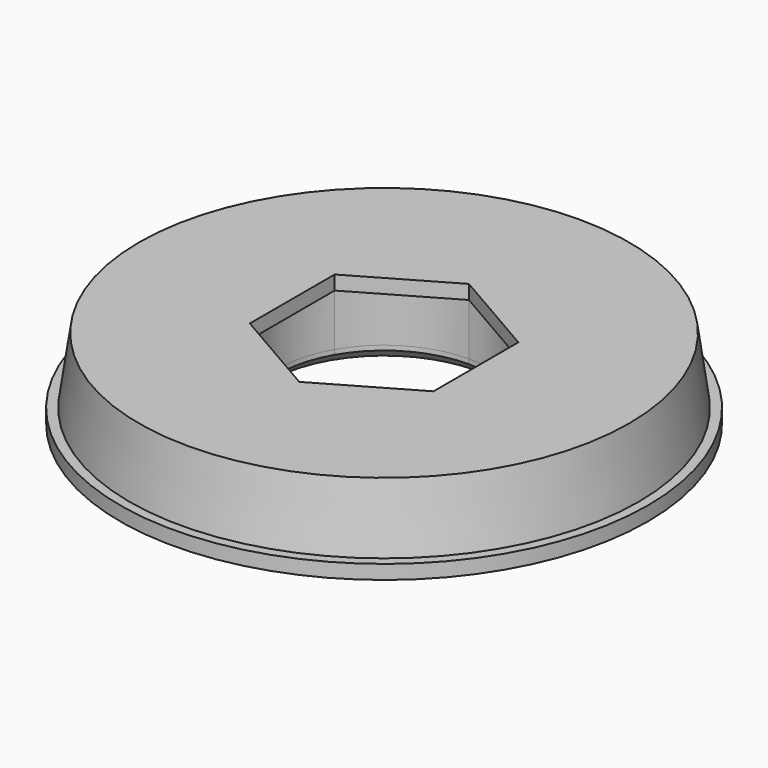
from build123d import *

# Parameters (mm, degrees)
F5_R          = 27
F6_DEPTH      = 7
F5_R_2        = 28
F7_DEPTH      = 1.5
F8_DEPTH      = 7.001
F8_DEPTH_BACK = 1.501
F9_DEPTH      = 5.5
F9_DEPTH_BACK = 1.501
F10_SIZE2     = 0.99999
F10_SIZE      = 6.99999
F11_SIZE      = 1


# Not quite as in the source:
# - a fillet or chamfer is up to 0.001 mm smaller than in the source, because OpenCascade refuses the exact size


with BuildPart() as f6:
    # F5 (on Top) → F6 (new body)
    with BuildSketch(Plane.XY):
        Circle(F5_R)
        with BuildLine():
            ThreePointArc((9.7427857926, 5.625), (10.8666655458, 2.9117142574), (11.25, 0))
            ThreePointArc((11.25, 0), (10.8666655458, -2.9117142574), (9.7427857926, -5.625))
            ThreePointArc((9.7427857926, -5.625), (5.625, -9.7427857926), (0, -11.25))
            ThreePointArc((0, -11.25), (-5.625, -9.7427857926), (-9.7427857926, -5.625))
            ThreePointArc((-9.7427857926, -5.625), (-11.25, 0), (-9.7427857926, 5.625))
            ThreePointArc((-9.7427857926, 5.625), (-5.625, 9.7427857926), (0, 11.25))
            ThreePointArc((0, 11.25), (5.625, 9.7427857926), (9.7427857926, 5.625))
        make_face(mode=Mode.SUBTRACT)
        with BuildLine():
            Line((-9.7427857926, -5.625), (-9.7427857926, 5.625))
            ThreePointArc((-9.7427857926, 5.625), (-11.25, 0), (-9.7427857926, -5.625))
        make_face()
        with BuildLine():
            Line((0, 11.25), (9.7427857926, 5.625))
            ThreePointArc((9.7427857926, 5.625), (5.625, 9.7427857926), (0, 11.25))
        make_face()
        with BuildLine():
            ThreePointArc((9.7427857926, -5.625), (10.8666655458, -2.9117142574), (11.25, 0))
            ThreePointArc((11.25, 0), (10.8666655458, 2.9117142574), (9.7427857926, 5.625))
            Line((9.7427857926, 5.625), (9.7427857926, -5.625))
        make_face()
        with BuildLine():
            ThreePointArc((0, -11.25), (5.625, -9.7427857926), (9.7427857926, -5.625))
            Line((9.7427857926, -5.625), (0, -11.25))
        make_face()
        with BuildLine():
            ThreePointArc((-9.7427857926, -5.625), (-5.625, -9.7427857926), (0, -11.25))
            Line((0, -11.25), (-9.7427857926, -5.625))
        make_face()
        with BuildLine():
            Line((-9.7427857926, 5.625), (0, 11.25))
            ThreePointArc((0, 11.25), (-5.625, 9.7427857926), (-9.7427857926, 5.625))
        make_face()
        Polygon((9.7427857926, -5.625), (9.7427857926, 5.625), (0, 11.25), (-9.7427857926, 5.625), (-9.7427857926, -5.625), (0, -11.25), align=None)
    extrude(amount=F6_DEPTH)

    # F5 (on Top) → F7 (join)
    with BuildSketch(Plane.XY):
        Circle(F5_R_2)
        Circle(F5_R, mode=Mode.SUBTRACT)
        Circle(F5_R)
        with BuildLine():
            ThreePointArc((9.7427857926, 5.625), (10.8666655458, 2.9117142574), (11.25, 0))
            ThreePointArc((11.25, 0), (10.8666655458, -2.9117142574), (9.7427857926, -5.625))
            ThreePointArc((9.7427857926, -5.625), (5.625, -9.7427857926), (0, -11.25))
            ThreePointArc((0, -11.25), (-5.625, -9.7427857926), (-9.7427857926, -5.625))
            ThreePointArc((-9.7427857926, -5.625), (-11.25, 0), (-9.7427857926, 5.625))
            ThreePointArc((-9.7427857926, 5.625), (-5.625, 9.7427857926), (0, 11.25))
            ThreePointArc((0, 11.25), (5.625, 9.7427857926), (9.7427857926, 5.625))
        make_face(mode=Mode.SUBTRACT)
        Polygon((9.7427857926, -5.625), (9.7427857926, 5.625), (0, 11.25), (-9.7427857926, 5.625), (-9.7427857926, -5.625), (0, -11.25), align=None)
        with BuildLine():
            ThreePointArc((9.7427857926, -5.625), (10.8666655458, -2.9117142574), (11.25, 0))
            ThreePointArc((11.25, 0), (10.8666655458, 2.9117142574), (9.7427857926, 5.625))
            Line((9.7427857926, 5.625), (9.7427857926, -5.625))
        make_face()
        with BuildLine():
            ThreePointArc((0, -11.25), (5.625, -9.7427857926), (9.7427857926, -5.625))
            Line((9.7427857926, -5.625), (0, -11.25))
        make_face()
        with BuildLine():
            ThreePointArc((-9.7427857926, -5.625), (-5.625, -9.7427857926), (0, -11.25))
            Line((0, -11.25), (-9.7427857926, -5.625))
        make_face()
        with BuildLine():
            Line((-9.7427857926, -5.625), (-9.7427857926, 5.625))
            ThreePointArc((-9.7427857926, 5.625), (-11.25, 0), (-9.7427857926, -5.625))
        make_face()
        with BuildLine():
            Line((0, 11.25), (9.7427857926, 5.625))
            ThreePointArc((9.7427857926, 5.625), (5.625, 9.7427857926), (0, 11.25))
        make_face()
        with BuildLine():
            Line((-9.7427857926, 5.625), (0, 11.25))
            ThreePointArc((0, 11.25), (-5.625, 9.7427857926), (-9.7427857926, 5.625))
        make_face()
    extrude(amount=-F7_DEPTH)

    # F5 (on Top) → F8 (cut, two sides)
    with BuildSketch(Plane.XY) as f8_sk:
        Polygon((9.7427857926, -5.625), (9.7427857926, 5.625), (0, 11.25), (-9.7427857926, 5.625), (-9.7427857926, -5.625), (0, -11.25), align=None)
    extrude(amount=F8_DEPTH, mode=Mode.SUBTRACT)
    extrude(f8_sk.sketch, amount=-F8_DEPTH_BACK, mode=Mode.SUBTRACT)

    # F5 (on Top) → F9 (cut, two sides)
    with BuildSketch(Plane.XY) as f9_sk:
        with BuildLine():
            ThreePointArc((-9.7427857926, -5.625), (-5.625, -9.7427857926), (0, -11.25))
            Line((0, -11.25), (-9.7427857926, -5.625))
        make_face()
        with BuildLine():
            ThreePointArc((0, -11.25), (5.625, -9.7427857926), (9.7427857926, -5.625))
            Line((9.7427857926, -5.625), (0, -11.25))
        make_face()
        with BuildLine():
            ThreePointArc((9.7427857926, -5.625), (10.8666655458, -2.9117142574), (11.25, 0))
            ThreePointArc((11.25, 0), (10.8666655458, 2.9117142574), (9.7427857926, 5.625))
            Line((9.7427857926, 5.625), (9.7427857926, -5.625))
        make_face()
        with BuildLine():
            Line((0, 11.25), (9.7427857926, 5.625))
            ThreePointArc((9.7427857926, 5.625), (5.625, 9.7427857926), (0, 11.25))
        make_face()
        with BuildLine():
            Line((-9.7427857926, 5.625), (0, 11.25))
            ThreePointArc((0, 11.25), (-5.625, 9.7427857926), (-9.7427857926, 5.625))
        make_face()
        with BuildLine():
            Line((-9.7427857926, -5.625), (-9.7427857926, 5.625))
            ThreePointArc((-9.7427857926, 5.625), (-11.25, 0), (-9.7427857926, -5.625))
        make_face()
    extrude(amount=F9_DEPTH, mode=Mode.SUBTRACT)
    extrude(f9_sk.sketch, amount=-F9_DEPTH_BACK, mode=Mode.SUBTRACT)

    # F10 (size 7 and 1 in the source; OpenCascade refuses exactly that, so slightly less here)
    f10_edges = [f6.edges().sort_by_distance(p)[0] for p in [
        (-27, 0, 7),
    ]]
    f10_side = f6.faces().sort_by_distance((-27, 0, 3.5))[0]
    chamfer(f10_edges, length=F10_SIZE, length2=F10_SIZE2, reference=f10_side)

    # F11
    f11_edges = [f6.edges().sort_by_distance(p)[0] for p in [
        (0, 11.25, -1.5),
    ]]
    chamfer(f11_edges, length=F11_SIZE)


solid = f6.part
